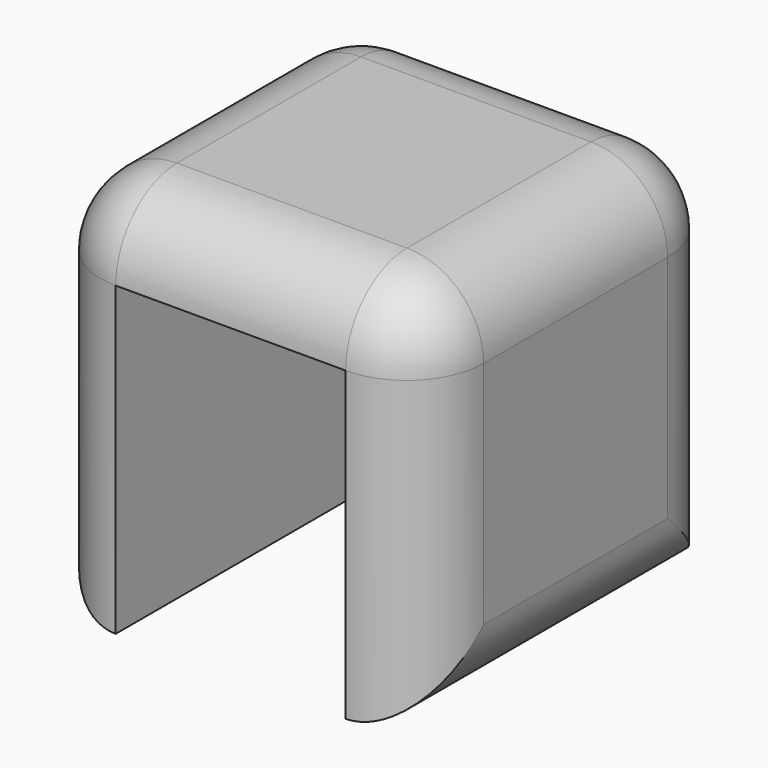
from build123d import *

# Parameters (mm, degrees)
F1_DEPTH = 25.4
F2_R     = 5.07999


# Not quite as in the source:
# - a fillet or chamfer is up to 0.001 mm smaller than in the source, because OpenCascade refuses the exact size


with BuildPart() as f1:
    # F0 (on Front) → F1 (new body)
    with BuildSketch(Plane.XZ):
        Polygon((25.4, 0), (0, 0), (0, -25.4), (5.08, -25.4), (5.08, -5.08), (20.32, -5.08), (20.32, -25.4), (25.4, -25.4), align=None)
    extrude(amount=F1_DEPTH)

    # F2 (radius 5.08 in the source; OpenCascade refuses exactly that, so slightly less here)
    f2_edges = [f1.edges().sort_by_distance(p)[0] for p in [
        (0, -12.7, 0),
        (12.7, -25.4, 0),
        (25.4, -12.7, 0),
        (12.7, 0, 0),
        (0, -25.4, -12.7),
        (0, 0, -12.7),
        (25.4, 0, -12.7),
        (25.4, -25.4, -12.7),
        (0, -12.7, -25.4),
        (25.4, -12.7, -25.4),
    ]]
    fillet(f2_edges, radius=F2_R)


solid = f1.part
